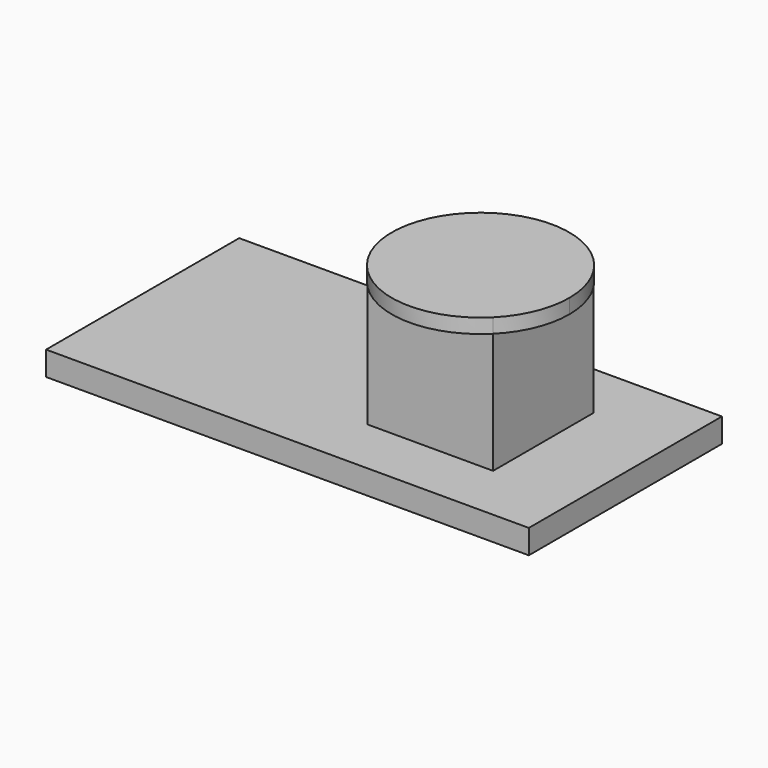
from build123d import *

# Parameters (mm, degrees)
F0_W     = 20
F0_H     = 12
F0_H_2   = 20
F0_W_2   = 17
F0_H_3   = 3
F0_W_3   = 3
F0_W_4   = 10.8891367149
F0_H_4   = 26
F1_DEPTH = 5
F2_DEPTH = 30
F4_DEPTH = 3


# Not quite as in the source:
# - a feature names something its author has since deleted; it is built from what else it names


with BuildPart() as f1:
    # F0 (on Top) → F1 (new body)
    with BuildSketch(Plane.XY):
        Polygon((-50, 25), (-50, -25), (-3.8891367149, -25), (-3.8891367149, -13), (-3.8891367149, 13), (-3.8891367149, 25), align=None)
        Polygon((-3.8891367149, -13), (-3.8891367149, -25), (10, -25), (10, -13), (7, -13), align=None)
        with Locations((20, -19)):
            Rectangle(F0_W, F0_H)
        Polygon((30, -13), (30, -25), (50, -25), (50, -13), (33, -13), align=None)
        Polygon((50, 25), (30, 25), (30, 13), (33, 13), (50, 13), align=None)
        with Locations((20, 0)):
            Rectangle(F0_W, F0_H_2)
        with Locations((41.5, 0)):
            Rectangle(F0_W_2, F0_H_2)
        with Locations((20, 19)):
            Rectangle(F0_W, F0_H)
        with Locations((20, 11.5)):
            Rectangle(F0_W, F0_H_3)
        with Locations((31.5, 11.5)):
            Rectangle(F0_W_3, F0_H_3)
        with Locations((41.5, 11.5)):
            Rectangle(F0_W_2, F0_H_3)
        with Locations((31.5, 0)):
            Rectangle(F0_W_3, F0_H_2)
        with Locations((41.5, -11.5)):
            Rectangle(F0_W_2, F0_H_3)
        with Locations((31.5, -11.5)):
            Rectangle(F0_W_3, F0_H_3)
        with Locations((20, -11.5)):
            Rectangle(F0_W, F0_H_3)
        with Locations((1.5554316426, 0)):
            Rectangle(F0_W_4, F0_H_4)
        Polygon((10, 25), (-3.8891367149, 25), (-3.8891367149, 13), (7, 13), (10, 13), align=None)
        Polygon((7, -13), (10, -13), (10, -10), (10, 10), (10, 13), (7, 13), align=None)
    extrude(amount=F1_DEPTH)

    # F0 (on Top) → F2 (join)
    with BuildSketch(Plane.XY):
        with Locations((20, 11.5)):
            Rectangle(F0_W, F0_H_3)
        with Locations((31.5, 11.5)):
            Rectangle(F0_W_3, F0_H_3)
        with Locations((31.5, 0)):
            Rectangle(F0_W_3, F0_H_2)
        with Locations((31.5, -11.5)):
            Rectangle(F0_W_3, F0_H_3)
        with Locations((20, -11.5)):
            Rectangle(F0_W, F0_H_3)
        Polygon((7, -13), (10, -13), (10, -10), (10, 10), (10, 13), (7, 13), align=None)
    extrude(amount=F2_DEPTH)

    # F3 (on face) → F4 (join)
    with BuildSketch(Plane.XY.offset(30)):
        with BuildLine():
            ThreePointArc((38.3847763109, 0), (36.9853185434, 7.0355493019), (33, 13))
            Line((33, 13), (20, 0))
            Line((20, 0), (33, -13))
            ThreePointArc((33, -13), (36.9853185434, -7.0355493019), (38.3847763109, 0))
        make_face()
        with BuildLine():
            Line((20, 0), (33, 13))
            ThreePointArc((33, 13), (20, 18.3847763109), (7, 13))
            Line((7, 13), (20, 0))
        make_face()
        with BuildLine():
            Line((33, -13), (20, 0))
            Line((20, 0), (7, -13))
            ThreePointArc((7, -13), (20, -18.3847763109), (33, -13))
        make_face()
        Polygon((7, -13), (20, 0), (7, 13), align=None)
        with BuildLine():
            Line((7, -13), (7, 13))
            ThreePointArc((7, 13), (1.6152236891, 0), (7, -13))
        make_face()
    extrude(amount=F4_DEPTH)


solid = f1.part
